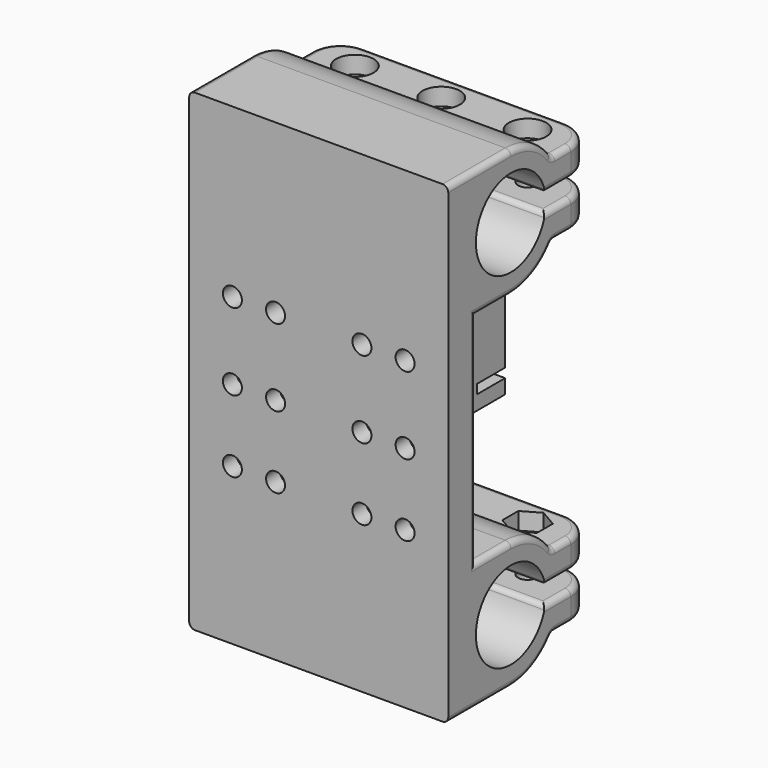
from build123d import *

# Parameters (mm, degrees)
F1_DEPTH               = 45
F2_R                   = 1
F4_DEPTH               = 7.6
F5_W                   = 43
F5_H                   = 12
F6_DEPTH               = 1.5
F8_DEPTH               = 3
F9_R                   = 1.65
F10_DEPTH              = 13.601
F13_D                  = 3.3
F13_DEPTH              = 14
F13_CBORE_D            = 6.5
F13_CBORE_DEPTH        = 3
F13_TIP                = 0.9914200214
F13_ON_F12_D           = 3.3
F13_ON_F12_DEPTH       = 14
F13_ON_F12_CBORE_D     = 6.5
F13_ON_F12_CBORE_DEPTH = 3
F13_ON_F12_TIP         = 0.9914200214
F15_DEPTH              = 3
F17_DEPTH              = 3
F18_R                  = 5
F19_R                  = 0.99999
F21_DEPTH              = 3
F22_R                  = 1.65
F23_DEPTH              = 6.001


# Not quite as in the source:
# - a fillet or chamfer is up to 0.001 mm smaller than in the source, because OpenCascade refuses the exact size


with BuildPart() as f1:
    # F0 (on Right) → F1 (new body)
    with BuildSketch(Plane.YZ):
        with BuildLine():
            Line((0, 82.2), (0, 0))
            Line((0, 0), (13.6, 0))
            ThreePointArc((13.6, 0), (18.6527220387, 1.2166807195), (22.5977775034, 4.6))
            Line((22.5977775034, 4.6), (31.6, 4.6))
            Line((31.6, 4.6), (31.6, 9.6))
            Line((31.6, 9.6), (21.0505033387, 9.6))
            ThreePointArc((21.0505033387, 9.6), (6, 11.1), (21.0505033387, 12.6))
            Line((21.0505033387, 12.6), (31.6, 12.6))
            Line((31.6, 12.6), (31.6, 17.6))
            Line((31.6, 17.6), (22.5977775034, 17.6))
            ThreePointArc((22.5977775034, 17.6), (18.6527220387, 20.9833192805), (13.6, 22.2))
            Line((13.6, 22.2), (6, 22.2))
            Line((6, 22.2), (6, 60))
            Line((6, 60), (13.6, 60))
            ThreePointArc((13.6, 60), (18.6527220387, 61.2166807195), (22.5977775034, 64.6))
            Line((22.5977775034, 64.6), (31.6, 64.6))
            Line((31.6, 64.6), (31.6, 69.6))
            Line((31.6, 69.6), (21.0505033387, 69.6))
            ThreePointArc((21.0505033387, 69.6), (6, 71.1), (21.0505033387, 72.6))
            Line((21.0505033387, 72.6), (31.6, 72.6))
            Line((31.6, 72.6), (31.6, 77.6000022888))
            Line((31.6, 77.6000022888), (22.5977758499, 77.6000022888))
            ThreePointArc((22.5977758499, 77.6000022888), (18.6527207816, 80.9833199231), (13.6, 82.2))
            Line((13.6, 82.2), (0, 82.2))
        make_face()
    extrude(amount=F1_DEPTH)

    # F2
    f2_edges = [f1.edges().sort_by_distance(p)[0] for p in [
        (0, 6, 41.1),
        (45, 6, 41.1),
    ]]
    fillet(f2_edges, radius=F2_R)

    # F3 (on face) → F4 (join)
    with BuildSketch(Plane(origin=(0, 6, 0), x_dir=(-1, 0, 0), z_dir=(0, 1, 0))):
        with BuildLine():
            Line((-28.75, 57.6), (-43.15, 57.6))
            Line((-43.15, 57.6), (-43.15, 58.55))
            ThreePointArc((-43.15, 58.55), (-42.5, 59.2), (-41.85, 58.55))
            ThreePointArc((-41.85, 58.55), (-41.8207106781, 58.4792893219), (-41.75, 58.45))
            Line((-41.75, 58.45), (-41.25, 58.45))
            ThreePointArc((-41.25, 58.45), (-41.1792893219, 58.4792893219), (-41.15, 58.55))
            ThreePointArc((-41.15, 58.55), (-40.5, 59.2), (-39.85, 58.55))
            ThreePointArc((-39.85, 58.55), (-39.8207106781, 58.4792893219), (-39.75, 58.45))
            Line((-39.75, 58.45), (-39.25, 58.45))
            ThreePointArc((-39.25, 58.45), (-39.1792893219, 58.4792893219), (-39.15, 58.55))
            ThreePointArc((-39.15, 58.55), (-38.5, 59.2), (-37.85, 58.55))
            ThreePointArc((-37.85, 58.55), (-37.8207106781, 58.4792893219), (-37.75, 58.45))
            Line((-37.75, 58.45), (-37.5, 58.45))
            Line((-37.5, 58.45), (-37.25, 58.45))
            ThreePointArc((-37.25, 58.45), (-37.1792893219, 58.4792893219), (-37.15, 58.55))
            ThreePointArc((-37.15, 58.55), (-36.5, 59.2), (-35.85, 58.55))
            ThreePointArc((-35.85, 58.55), (-35.8207106781, 58.4792893219), (-35.75, 58.45))
            Line((-35.75, 58.45), (-35.25, 58.45))
            ThreePointArc((-35.25, 58.45), (-35.1792893219, 58.4792893219), (-35.15, 58.55))
            ThreePointArc((-35.15, 58.55), (-34.5, 59.2), (-33.85, 58.55))
            ThreePointArc((-33.85, 58.55), (-33.8207106781, 58.4792893219), (-33.75, 58.45))
            Line((-33.75, 58.45), (-33.25, 58.45))
            ThreePointArc((-33.25, 58.45), (-33.1792893219, 58.4792893219), (-33.15, 58.55))
            ThreePointArc((-33.15, 58.55), (-32.5, 59.2), (-31.85, 58.55))
            ThreePointArc((-31.85, 58.55), (-31.8207106781, 58.4792893219), (-31.75, 58.45))
            Line((-31.75, 58.45), (-31.5, 58.45))
            Line((-31.5, 58.45), (-31.25, 58.45))
            ThreePointArc((-31.25, 58.45), (-31.1792893219, 58.4792893219), (-31.15, 58.55))
            ThreePointArc((-31.15, 58.55), (-30.5, 59.2), (-29.85, 58.55))
            ThreePointArc((-29.85, 58.55), (-29.8207106781, 58.4792893219), (-29.75, 58.45))
            Line((-29.75, 58.45), (-29.25, 58.45))
            ThreePointArc((-29.25, 58.45), (-29.1792893219, 58.4792893219), (-29.15, 58.55))
            ThreePointArc((-29.15, 58.55), (-28.5, 59.2), (-27.85, 58.55))
            ThreePointArc((-27.85, 58.55), (-27.8207106781, 58.4792893219), (-27.75, 58.45))
            Line((-27.75, 58.45), (-27.25, 58.45))
            ThreePointArc((-27.25, 58.45), (-27.1792893219, 58.4792893219), (-27.15, 58.55))
            ThreePointArc((-27.15, 58.55), (-26.5, 59.2), (-25.85, 58.55))
            ThreePointArc((-25.85, 58.55), (-25.8207106781, 58.4792893219), (-25.75, 58.45))
            Line((-25.75, 58.45), (-25.5, 58.45))
            Line((-25.5, 58.45), (-25.25, 58.45))
            ThreePointArc((-25.25, 58.45), (-25.1792893219, 58.4792893219), (-25.15, 58.55))
            ThreePointArc((-25.15, 58.55), (-24.5, 59.2), (-23.85, 58.55))
            ThreePointArc((-23.85, 58.55), (-23.8207106781, 58.4792893219), (-23.75, 58.45))
            Line((-23.75, 58.45), (-23.25, 58.45))
            ThreePointArc((-23.25, 58.45), (-23.1792893219, 58.4792893219), (-23.15, 58.55))
            ThreePointArc((-23.15, 58.55), (-22.5, 59.2), (-21.85, 58.55))
            ThreePointArc((-21.85, 58.55), (-21.8207106781, 58.4792893219), (-21.75, 58.45))
            Line((-21.75, 58.45), (-21.25, 58.45))
            ThreePointArc((-21.25, 58.45), (-21.1792893219, 58.4792893219), (-21.15, 58.55))
            ThreePointArc((-21.15, 58.55), (-20.5, 59.2), (-19.85, 58.55))
            ThreePointArc((-19.85, 58.55), (-19.8207106781, 58.4792893219), (-19.75, 58.45))
            Line((-19.75, 58.45), (-19.5, 58.45))
            Line((-19.5, 58.45), (-19.25, 58.45))
            ThreePointArc((-19.25, 58.45), (-19.1792893219, 58.4792893219), (-19.15, 58.55))
            ThreePointArc((-19.15, 58.55), (-18.5, 59.2), (-17.85, 58.55))
            ThreePointArc((-17.85, 58.55), (-17.8207106781, 58.4792893219), (-17.75, 58.45))
            Line((-17.75, 58.45), (-17.25, 58.45))
            ThreePointArc((-17.25, 58.45), (-17.1792893219, 58.4792893219), (-17.15, 58.55))
            ThreePointArc((-17.15, 58.55), (-16.5, 59.2), (-15.85, 58.55))
            ThreePointArc((-15.85, 58.55), (-15.8207106781, 58.4792893219), (-15.75, 58.45))
            Line((-15.75, 58.45), (-15.25, 58.45))
            ThreePointArc((-15.25, 58.45), (-15.1792893219, 58.4792893219), (-15.15, 58.55))
            ThreePointArc((-15.15, 58.55), (-14.5, 59.2), (-13.85, 58.55))
            ThreePointArc((-13.85, 58.55), (-13.8207106781, 58.4792893219), (-13.75, 58.45))
            Line((-13.75, 58.45), (-13.5, 58.45))
            Line((-13.5, 58.45), (-13.25, 58.45))
            ThreePointArc((-13.25, 58.45), (-13.1792893219, 58.4792893219), (-13.15, 58.55))
            ThreePointArc((-13.15, 58.55), (-12.5, 59.2), (-11.85, 58.55))
            ThreePointArc((-11.85, 58.55), (-11.8207106781, 58.4792893219), (-11.75, 58.45))
            Line((-11.75, 58.45), (-11.25, 58.45))
            ThreePointArc((-11.25, 58.45), (-11.1792893219, 58.4792893219), (-11.15, 58.55))
            ThreePointArc((-11.15, 58.55), (-10.5, 59.2), (-9.85, 58.55))
            ThreePointArc((-9.85, 58.55), (-9.8207106781, 58.4792893219), (-9.75, 58.45))
            Line((-9.75, 58.45), (-9.25, 58.45))
            ThreePointArc((-9.25, 58.45), (-9.1792893219, 58.4792893219), (-9.15, 58.55))
            ThreePointArc((-9.15, 58.55), (-8.5, 59.2), (-7.85, 58.55))
            ThreePointArc((-7.85, 58.55), (-7.8207106781, 58.4792893219), (-7.75, 58.45))
            Line((-7.75, 58.45), (-7.5, 58.45))
            Line((-7.5, 58.45), (-7.25, 58.45))
            ThreePointArc((-7.25, 58.45), (-7.1792893219, 58.4792893219), (-7.15, 58.55))
            ThreePointArc((-7.15, 58.55), (-6.5, 59.2), (-5.85, 58.55))
            ThreePointArc((-5.85, 58.55), (-5.8207106781, 58.4792893219), (-5.75, 58.45))
            Line((-5.75, 58.45), (-5.25, 58.45))
            ThreePointArc((-5.25, 58.45), (-5.1792893219, 58.4792893219), (-5.15, 58.55))
            ThreePointArc((-5.15, 58.55), (-4.5, 59.2), (-3.85, 58.55))
            ThreePointArc((-3.85, 58.55), (-3.8207106781, 58.4792893219), (-3.75, 58.45))
            Line((-3.75, 58.45), (-3.25, 58.45))
            ThreePointArc((-3.25, 58.45), (-3.1792893219, 58.4792893219), (-3.15, 58.55))
            ThreePointArc((-3.15, 58.55), (-2.5, 59.2), (-1.85, 58.55))
            Line((-1.85, 58.55), (-1.85, 57.6))
            Line((-1.85, 57.6), (-16.25, 57.6))
            ThreePointArc((-16.25, 57.6), (-20.75, 53.1), (-16.25, 48.6))
            Line((-16.25, 48.6), (-1, 48.6))
            Line((-1, 48.6), (-1, 60))
            Line((-1, 60), (-44, 60))
            Line((-44, 60), (-44, 48.6))
            Line((-44, 48.6), (-28.75, 48.6))
            ThreePointArc((-28.75, 48.6), (-24.25, 53.1), (-28.75, 57.6))
        make_face()
        with BuildLine():
            Line((-28.75, 47), (-44, 47))
            Line((-44, 47), (-44, 44.5))
            Line((-44, 44.5), (-1, 44.5))
            Line((-1, 44.5), (-1, 47))
            Line((-1, 47), (-16.25, 47))
            ThreePointArc((-16.25, 47), (-19.5651685427, 47.9794865947), (-21.8156934307, 50.6033909726))
            ThreePointArc((-21.8156934307, 50.6033909726), (-22.5, 51.0464308462), (-23.1843065693, 50.6033909726))
            ThreePointArc((-23.1843065693, 50.6033909726), (-25.4348314573, 47.9794865947), (-28.75, 47))
        make_face()
    extrude(amount=F4_DEPTH)

    # F5 (on face) → F6 (join)
    with BuildSketch(Plane(origin=(0, 6, 0), x_dir=(-1, 0, 0), z_dir=(0, 1, 0))):
        with Locations((-22.5, 53)):
            Rectangle(F5_W, F5_H)
    extrude(amount=F6_DEPTH)

    # F7 (on face) → F8 (cut)
    with BuildSketch(Plane(origin=(0, 13.6, 0), x_dir=(-1, 0, 0), z_dir=(0, 1, 0))):
        Polygon((-9.2320508076, 50.1), (-5.7679491924, 50.1), (-4.0358983849, 53.1), (-5.7679491924, 56.1), (-9.2320508076, 56.1), (-10.9641016151, 53.1), align=None)
        Polygon((-39.2320508076, 50.1), (-35.7679491924, 50.1), (-34.0358983849, 53.1), (-35.7679491924, 56.1), (-39.2320508076, 56.1), (-40.9641016151, 53.1), align=None)
        Polygon((-31.7320508076, 50.1), (-28.2679491924, 50.1), (-26.5358983849, 53.1), (-28.2679491924, 56.1), (-31.7320508076, 56.1), (-33.4641016151, 53.1), align=None)
        Polygon((-16.7320508076, 50.1), (-13.2679491924, 50.1), (-11.5358983849, 53.1), (-13.2679491924, 56.1), (-16.7320508076, 56.1), (-18.4641016151, 53.1), align=None)
    extrude(amount=-F8_DEPTH, mode=Mode.SUBTRACT)

    # F9 (on face) → F10 (cut, through all)
    with BuildSketch(Plane(origin=(0, 13.6, 0), x_dir=(-1, 0, 0), z_dir=(0, 1, 0))):
        with Locations((-37.5, 53.1)):
            Circle(F9_R)
        with Locations((-7.5, 53.1)):
            Circle(F9_R)
        with Locations((-30, 53.1)):
            Circle(F9_R)
        with Locations((-15, 53.1)):
            Circle(F9_R)
    extrude(amount=-F10_DEPTH, mode=Mode.SUBTRACT)

    # F13
    with Locations(Plane.XY.offset(77.6000022888)):
        with Locations((7.5, 26.6), (37.5, 26.6), (22.5, 26.6)):
            CounterBoreHole(F13_D / 2, F13_CBORE_D / 2, F13_CBORE_DEPTH, depth=F13_DEPTH)
            with Locations((0, 0, -(F13_DEPTH + F13_TIP / 2))):  # 118° drill point
                Cone(0, F13_D / 2, F13_TIP, mode=Mode.SUBTRACT)

    # F13 on F12
    with Locations(Plane(origin=(0, 0, 4.6), x_dir=(1, 0, 0), z_dir=(0, 0, -1))):
        with Locations((37.5, -26.6), (7.5, -26.6), (22.5, -26.6)):
            CounterBoreHole(F13_ON_F12_D / 2, F13_ON_F12_CBORE_D / 2, F13_ON_F12_CBORE_DEPTH, depth=F13_ON_F12_DEPTH)
            with Locations((0, 0, -(F13_ON_F12_DEPTH + F13_ON_F12_TIP / 2))):  # 118° drill point
                Cone(0, F13_ON_F12_D / 2, F13_ON_F12_TIP, mode=Mode.SUBTRACT)

    # F14 (on face) → F15 (cut)
    with BuildSketch(Plane.XY.offset(17.6)):
        Polygon((4.5, 28.3320508076), (4.5, 24.8679491924), (7.5, 23.1358983849), (10.5, 24.8679491924), (10.5, 28.3320508076), (7.5, 30.0641016151), align=None)
        Polygon((34.5, 28.3320508076), (34.5, 24.8679491924), (37.5, 23.1358983849), (40.5, 24.8679491924), (40.5, 28.3320508076), (37.5, 30.0641016151), align=None)
        Polygon((25.5, 24.8679491924), (25.5, 28.3320508076), (22.5, 30.0641016151), (19.5, 28.3320508076), (19.5, 24.8679491924), (22.5, 23.1358983849), align=None)
    extrude(amount=-F15_DEPTH, mode=Mode.SUBTRACT)

    # F16 (on face) → F17 (cut)
    with BuildSketch(Plane(origin=(0, 0, 64.6), x_dir=(1, 0, 0), z_dir=(0, 0, -1))):
        Polygon((34.5, -24.8679491924), (34.5, -28.3320508076), (37.5, -30.0641016151), (40.5, -28.3320508076), (40.5, -24.8679491924), (37.5, -23.1358983849), align=None)
        Polygon((4.5, -24.8679491924), (4.5, -28.3320508076), (7.5, -30.0641016151), (10.5, -28.3320508076), (10.5, -24.8679491924), (7.5, -23.1358983849), align=None)
        Polygon((19.5, -24.8679491924), (19.5, -28.3320508076), (22.5, -30.0641016151), (25.5, -28.3320508076), (25.5, -24.8679491924), (22.5, -23.1358983849), align=None)
    extrude(amount=-F17_DEPTH, mode=Mode.SUBTRACT)

    # F18
    f18_edges = [f1.edges().sort_by_distance(p)[0] for p in [
        (0, 31.6, 67.1),
        (0, 31.6, 75.100001),
        (0, 31.6, 15.1),
        (0, 31.6, 7.1),
        (45, 31.6, 7.1),
        (45, 31.6, 15.1),
        (45, 31.6, 67.1),
        (45, 31.6, 75.100001),
    ]]
    fillet(f18_edges, radius=F18_R)

    # F19 (radius 1 in the source; OpenCascade refuses exactly that, so slightly less here)
    f19_edges = [f1.edges().sort_by_distance(p)[0] for p in [
        (22.5, 22.597778, 64.6),
        (22.5, 21.050503, 72.6),
        (22.5, 21.050503, 69.6),
        (22.5, 22.597776, 77.600002),
        (22.5, 22.597778, 17.6),
        (22.5, 21.050503, 9.6),
        (22.5, 21.050503, 12.6),
        (22.5, 22.597778, 4.6),
        (0, 6.8, 0),
        (0, 6.8, 82.2),
        (0, 9.3, 60),
        (0, 9.3, 22.2),
        (0, 23.825252, 12.6),
        (0, 23.825252, 9.6),
        (0, 23.825252, 69.6),
        (0, 23.825252, 72.6),
        (0, 24.598889, 64.6),
        (0, 18.652722, 61.216681),
        (0, 18.652722, 20.983319),
        (0, 24.598888, 77.600002),
        (0, 24.598889, 17.6),
        (0, 18.652721, 80.98332),
        (0, 18.652722, 1.216681),
        (0, 24.598889, 4.6),
        (1.464466, 30.135534, 64.6),
        (22.5, 31.6, 64.6),
        (45, 24.598889, 64.6),
        (43.535534, 30.135534, 64.6),
        (1.464466, 30.135534, 69.6),
        (45, 18.652722, 61.216681),
        (22.5, 31.6, 69.6),
        (43.535534, 30.135534, 69.6),
        (45, 23.825252, 69.6),
        (1.464466, 30.135534, 72.6),
        (22.5, 31.6, 72.6),
        (45, 23.825252, 72.6),
        (43.535534, 30.135534, 72.6),
        (45, 9.3, 22.2),
        (1.464466, 30.135534, 77.600002),
        (45, 18.652722, 20.983319),
        (22.5, 31.6, 77.600002),
        (43.535534, 30.135534, 77.600002),
        (45, 24.598888, 77.600002),
        (22.5, 31.6, 17.6),
        (1.464466, 30.135534, 17.6),
        (43.535534, 30.135534, 17.6),
        (45, 24.598889, 17.6),
        (45, 18.652721, 80.98332),
        (1.464466, 30.135534, 12.6),
        (45, 6.8, 82.2),
        (22.5, 31.6, 12.6),
        (45, 23.825252, 12.6),
        (43.535534, 30.135534, 12.6),
        (45, 6.8, 0),
        (22.5, 31.6, 9.6),
        (1.464466, 30.135534, 9.6),
        (43.535534, 30.135534, 9.6),
        (45, 23.825252, 9.6),
        (45, 18.652722, 1.216681),
        (1.464466, 30.135534, 4.6),
        (22.5, 31.6, 4.6),
        (45, 24.598889, 4.6),
        (43.535534, 30.135534, 4.6),
        (45, 9.3, 60),
    ]]
    fillet(f19_edges, radius=F19_R)

    # F20 (on face) → F21 (cut)
    with BuildSketch(Plane(origin=(0, 6, 0), x_dir=(-1, 0, 0), z_dir=(0, 1, 0))):
        Polygon((-35.7679491924, 42.7), (-39.2320508076, 42.7), (-40.9641016151, 39.7), (-39.2320508076, 36.7), (-35.7679491924, 36.7), (-34.0358983849, 39.7), align=None)
        Polygon((-28.2679491924, 42.7), (-31.7320508076, 42.7), (-33.4641016151, 39.7), (-31.7320508076, 36.7), (-28.2679491924, 36.7), (-26.5358983849, 39.7), align=None)
        Polygon((-13.2679491924, 42.7), (-16.7320508076, 42.7), (-18.4641016151, 39.7), (-16.7320508076, 36.7), (-13.2679491924, 36.7), (-11.5358983849, 39.7), align=None)
        Polygon((-5.7679491924, 42.7), (-9.2320508076, 42.7), (-10.9641016151, 39.7), (-9.2320508076, 36.7), (-5.7679491924, 36.7), (-4.0358983849, 39.7), align=None)
        Polygon((-39.2320508076, 24.2), (-35.7679491924, 24.2), (-34.0358983849, 27.2), (-35.7679491924, 30.2), (-39.2320508076, 30.2), (-40.9641016151, 27.2), align=None)
        Polygon((-31.7320508076, 24.2), (-28.2679491924, 24.2), (-26.5358983849, 27.2), (-28.2679491924, 30.2), (-31.7320508076, 30.2), (-33.4641016151, 27.2), align=None)
        Polygon((-16.7320508076, 24.2), (-13.2679491924, 24.2), (-11.5358983849, 27.2), (-13.2679491924, 30.2), (-16.7320508076, 30.2), (-18.4641016151, 27.2), align=None)
        Polygon((-9.2320508076, 24.2), (-5.7679491924, 24.2), (-4.0358983849, 27.2), (-5.7679491924, 30.2), (-9.2320508076, 30.2), (-10.9641016151, 27.2), align=None)
    extrude(amount=-F21_DEPTH, mode=Mode.SUBTRACT)

    # F22 (on face) → F23 (cut, through all)
    with BuildSketch(Plane(origin=(0, 6, 0), x_dir=(-1, 0, 0), z_dir=(0, 1, 0))):
        with Locations((-37.5, 39.7)):
            Circle(F22_R)
        with Locations((-30, 39.7)):
            Circle(F22_R)
        with Locations((-15, 39.7)):
            Circle(F22_R)
        with Locations((-7.5, 39.7)):
            Circle(F22_R)
        with Locations((-7.5, 27.2)):
            Circle(F22_R)
        with Locations((-15, 27.2)):
            Circle(F22_R)
        with Locations((-30, 27.2)):
            Circle(F22_R)
        with Locations((-37.5, 27.2)):
            Circle(F22_R)
    extrude(amount=-F23_DEPTH, mode=Mode.SUBTRACT)


solid = f1.part
